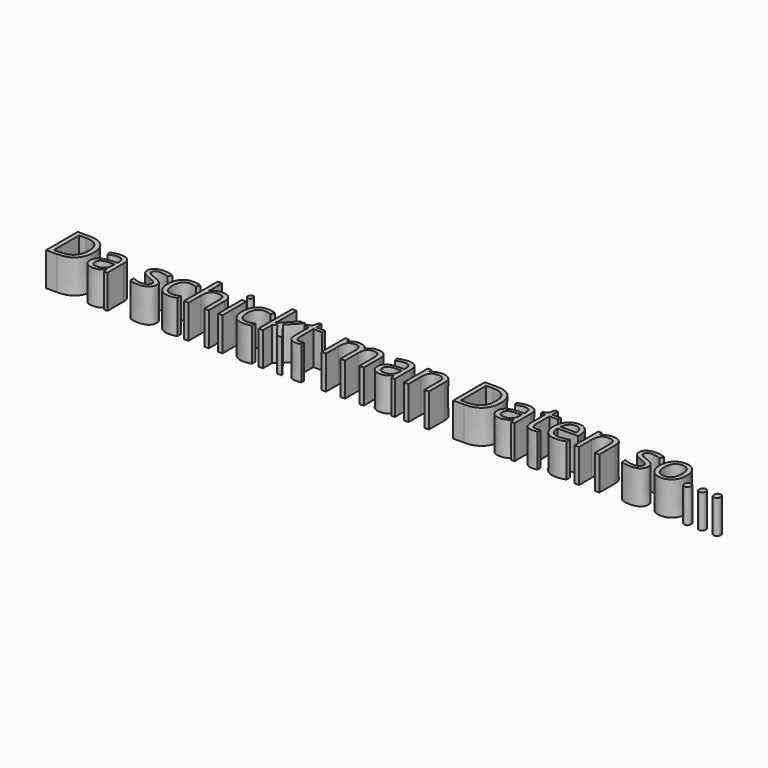
from build123d import *

# Parameters (mm, degrees)
F0_TEXT_SIZE = 41.9920620819
F1_DEPTH     = 25.4


# Not quite as in the source:
# - Text() gives the source's letters only with a copy of the font that has no kerning and outlines rounded to 1/6400 em; it was checked with that copy


with BuildPart() as f1:
    # F0 (on Top) → F1 (new body)
    with BuildSketch(Plane.XY):
        with Locations((-204.5532166958, -66.3853362203)):
            Text('Da schickt man Daten so...', F0_TEXT_SIZE, font='Open Sans', text_align=(TextAlign.LEFT, TextAlign.BOTTOM))
    extrude(amount=F1_DEPTH)


solid = f1.part
